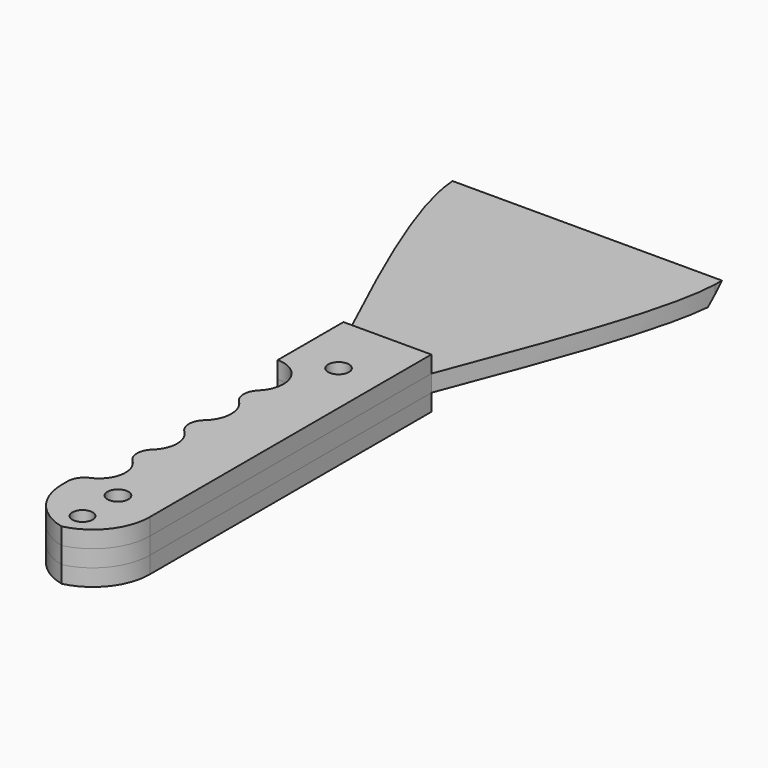
from build123d import *

# Parameters (mm, degrees)
F0_W         = 26.0835690424
F0_H         = 121.3984042406
F1_DEPTH     = 5
F2_T1_DEPTH  = 89.4974746831
F4_DEPTH     = 25
F5_T1_DEPTH  = 24.9013657706
F6_R         = 4.99999
F7_R         = 5
F8_T1_DEPTH  = 25.0040742563
F9_R         = 4.99999
F10_T1_DEPTH = 25.1951935832
F11_R        = 4.99999
F13_DEPTH    = 5
F15_DEPTH    = 5
F16_R        = 3.1
F17_DEPTH    = 25
F18_R        = 3
F19_DEPTH    = 25
F20_SIZE     = 4.99999


# Not quite as in the source:
# - a fillet or chamfer that OpenCascade refuses, or shapes differently, is made with other operations: its cross-section is extruded or revolved along the edge and cut away or added
# - a fillet or chamfer is up to 0.001 mm smaller than in the source, because OpenCascade refuses the exact size


with BuildPart() as f1:
    # F0 (on Top) → F1 (new body)
    with BuildSketch(Plane.XY):
        with BuildLine():
            Line((35.9049700201, 124.7347638011), (-44.0950299799, 124.7347638011))
            add(Edge.make_bspline(
                [(-13.5923651978, 46.1331680417), (-28.3171912792, 77.6195773739), (-43.0420173606, 109.1059867062), (-44.0950299799, 124.7347638011)],
                knots=[0, 0, 0, 0, 0.7080270969, 0.7080270969, 0.7080270969, 0.7080270969], degree=3))
            Line((-13.5923651978, 46.1331680417), (12.4912038445, 46.1331680417))
            add(Edge.make_bspline(
                [(12.4912038445, 46.1331680417), (23.8952472444, 75.9274680411), (35.2992906443, 105.7217680404), (35.9049700201, 122.1449805606)],
                knots=[0, 0, 0, 0, 0.6592241064, 0.6592241064, 0.6592241064, 0.6592241064], degree=3))
            Line((35.9049700201, 122.1449805606), (35.9049700201, 124.7347638011))
        make_face()
        with Locations((-0.5505806766, -14.5660340786)):
            Rectangle(F0_W, F0_H)
    extrude(amount=F1_DEPTH)

    # F2: fillet of radius 16.8994949366 on 2 edges, made by hand

    # F2_s2 → F2_t1 (cut)
    with BuildSketch(Plane.XY.offset(-42.2487373415)):
        with BuildLine():
            ThreePointArc((-13.5923651978, -58.3657412623), (-8.6426177295, -70.3154887306), (3.3071297388, -75.2652361989))
            Line((3.3071297388, -75.2652361989), (-13.5923651978, -75.2652361989))
            Line((-13.5923651978, -75.2652361989), (-13.5923651978, -58.3657412623))
        make_face()
        with BuildLine():
            ThreePointArc((-4.4082910921, -75.2652361989), (7.5414563762, -70.3154887306), (12.4912038445, -58.3657412623))
            Line((12.4912038445, -58.3657412623), (12.4912038445, -75.2652361989))
            Line((12.4912038445, -75.2652361989), (-4.4082910921, -75.2652361989))
        make_face()
    extrude(amount=F2_T1_DEPTH, mode=Mode.SUBTRACT)

    # F3 (on face) → F4 (cut)
    with BuildSketch(Plane.XY.offset(5)):
        with BuildLine():
            ThreePointArc((-13.5923651978, -52.2482340587), (-8.0995257077, -49.9730254459), (-5.8243170949, -44.4801859558))
            ThreePointArc((-5.8243170949, -44.4801859558), (-8.0995257077, -38.9873464656), (-13.5923651978, -36.7121378529))
            Line((-13.5923651978, -36.7121378529), (-13.5923651978, -52.2482340587))
        make_face()
        with BuildLine():
            Line((-13.5923651978, -17.6161278137), (-13.5923651978, -33.6357008568))
            ThreePointArc((-13.5923651978, -33.6357008568), (-7.9285908326, -31.2896887005), (-5.5825786763, -25.6259143353))
            ThreePointArc((-5.5825786763, -25.6259143353), (-7.9285908326, -19.96213997), (-13.5923651978, -17.6161278137))
        make_face()
        with BuildLine():
            Line((-13.5923651978, 2.3720021674), (-13.5923651978, -14.604575388))
            ThreePointArc((-13.5923651978, -14.604575388), (-7.5902386425, -12.1184131657), (-5.1040764201, -6.1162866103))
            ThreePointArc((-5.1040764201, -6.1162866103), (-7.5902386425, -0.1141600549), (-13.5923651978, 2.3720021674))
        make_face()
        with BuildLine():
            Line((-13.5923651978, 21.7131827375), (-13.5923651978, 4.5183054754))
            ThreePointArc((-13.5923651978, 4.5183054754), (-7.513058041, 7.0364369496), (-4.9949265668, 13.1157441065))
            ThreePointArc((-4.9949265668, 13.1157441065), (-7.513058041, 19.1950512633), (-13.5923651978, 21.7131827375))
        make_face()
    extrude(amount=-F4_DEPTH, mode=Mode.SUBTRACT)

    # F5: fillet of radius 5 on 1 edges, made by hand

    # F5_s2 → F5_t1 (cut)
    with BuildSketch(Plane.XY.offset(-9.9506828853)):
        with BuildLine():
            ThreePointArc((-10.5503778712, -37.3325370812), (-12.7631003469, -35.4895754009), (-13.5923651978, -32.7318646987))
            Line((-13.5923651978, -32.7318646987), (-13.5923651978, -36.7121378529))
            ThreePointArc((-13.5923651978, -36.7121378529), (-12.0400619013, -36.8688177604), (-10.5503778712, -37.3325370812))
        make_face()
    extrude(amount=F5_T1_DEPTH, mode=Mode.SUBTRACT)

    # F6 (radius 5 in the source; OpenCascade refuses exactly that, so slightly less here)
    f6_edges = [f1.edges().sort_by_distance(p)[0] for p in [
        (-13.510072, -33.635278, 2.5),
    ]]
    fillet(f6_edges, radius=F6_R)

    # F7
    f7_edges = [f1.edges().sort_by_distance(p)[0] for p in [
        (-13.592365, -52.248234, 2.5),
    ]]
    fillet(f7_edges, radius=F7_R)

    # F8: fillet of radius 5 on 1 edges, made by hand

    # F8_s2 → F8_t1 (cut)
    with BuildSketch(Plane.XY.offset(-10.0020371281)):
        with BuildLine():
            ThreePointArc((-10.5139954997, -18.2313000706), (-12.7521819912, -16.3894658503), (-13.5923651978, -13.6153129624))
            Line((-13.5923651978, -13.6153129624), (-13.5923651978, -17.6161278137))
            ThreePointArc((-13.5923651978, -17.6161278137), (-12.0227476565, -17.7714263892), (-10.5139954997, -18.2313000706))
        make_face()
    extrude(amount=F8_T1_DEPTH, mode=Mode.SUBTRACT)

    # F9 (radius 5 in the source; OpenCascade refuses exactly that, so slightly less here)
    f9_edges = [f1.edges().sort_by_distance(p)[0] for p in [
        (-13.49364, -14.604001, 2.5),
    ]]
    fillet(f9_edges, radius=F9_R)

    # F10: fillet of radius 5 on 1 edges, made by hand

    # F10_s2 → F10_t1 (cut)
    with BuildSketch(Plane.XY.offset(-10.0975967916)):
        with BuildLine():
            ThreePointArc((-10.4458249222, 1.7672614911), (-12.7316464532, 3.6063393511), (-13.5923651978, 6.411040884))
            Line((-13.5923651978, 6.411040884), (-13.5923651978, 2.3720021674))
            ThreePointArc((-13.5923651978, 2.3720021674), (-11.9903019195, 2.2194460885), (-10.4458249222, 1.7672614911))
        make_face()
    extrude(amount=F10_T1_DEPTH, mode=Mode.SUBTRACT)

    # F11 (radius 5 in the source; OpenCascade refuses exactly that, so slightly less here)
    f11_edges = [f1.edges().sort_by_distance(p)[0] for p in [
        (-13.223505, 4.526222, 2.5),
    ]]
    fillet(f11_edges, radius=F11_R)


with BuildPart() as f13:
    # F12 (on face) → F13 (new body)
    with BuildSketch(Plane.XY.offset(5)):
        with BuildLine():
            Line((12.4912038445, 46.1331680417), (-13.5923651978, 46.1331680417))
            Line((-13.5923651978, 46.1331680417), (-13.5923651978, 21.7131827375))
            ThreePointArc((-13.5923651978, 21.7131827375), (-5.6360261058, 16.3734456378), (-7.5628070571, 6.9870917553))
            add(Edge.make_bspline(
                [(-7.5911831215, -0.1132157245), (-7.7220544685, 0.0176144451), (-7.8479195294, 0.1550609527), (-7.9682435575, 0.2988565059), (-8.0825261727, 0.4486782277), (-8.1903056088, 0.604149631), (-8.3630630632, 0.8793988488), (-8.4314461626, 0.9966100443), (-8.4961606332, 1.1163214136), (-8.55706797, 1.2383679343), (-8.6140427893, 1.3625743295), (-8.7044044674, 1.5779889308), (-8.7398133996, 1.6682105076), (-8.7731600497, 1.7593543582), (-8.8044085072, 1.8513531954), (-8.8335265261, 1.9441378845), (-8.9259779929, 2.2647792954), (-8.9787300974, 2.4961463602), (-9.0183300846, 2.7307113036), (-9.0445030419, 2.9674123507), (-9.0571126109, 3.2051609509), (-9.0548218016, 3.7783711923), (-9.026462459, 4.1138191158), (-8.9710875527, 4.4460377153), (-8.889295394, 4.7719952295), (-8.7821710769, 5.0888005386), (-8.5974297226, 5.5195243383), (-8.5394639684, 5.6432713787), (-8.4775830857, 5.7648271817), (-8.4119138552, 5.8840174782), (-8.3425960964, 6.0006783584), (-8.1676441529, 6.274537971), (-8.0586255102, 6.4291429504), (-7.9431490529, 6.5780464502), (-7.8216795416, 6.7208756862), (-7.6947199209, 6.8573117912), (-7.5628070571, 6.9870917553)],
                knots=[0, 0, 0, 0, 0, 0, 0, 0.1452743272, 0.1452743272, 0.1452743272, 0.1452743272, 0.1452743272, 0.2488388047, 0.2488388047, 0.2488388047, 0.2488388047, 0.2488388047, 0.3220786555, 0.3220786555, 0.3220786555, 0.3220786555, 0.3220786555, 0.5000028667, 0.5000028667, 0.5000028667, 0.5000028667, 0.5000028667, 0.7511611873, 0.7511611873, 0.7511611873, 0.7511611873, 0.7511611873, 0.8547256681, 0.8547256681, 0.8547256681, 0.8547256681, 0.8547256681, 1, 1, 1, 1, 1, 1, 1], degree=6))
            ThreePointArc((-7.5911831215, -0.1132157245), (-5.1076987518, -6.3642415925), (-7.9519916275, -12.4595690698))
            add(Edge.make_bspline(
                [(-8.0741915729, -19.8201895772), (-8.2146874054, -19.6866523481), (-8.3498787146, -19.5457164219), (-8.4791425882, -19.397673153), (-8.6018965999, -19.242880944), (-8.7176036899, -19.0817628218), (-8.9020469019, -18.7970862585), (-8.9745726364, -18.6764633987), (-9.0431838813, -18.5531050443), (-9.1077251179, -18.4271925476), (-9.1680556762, -18.2989190025), (-9.2641399851, -18.0751050196), (-9.3020074648, -17.9806151083), (-9.3376061459, -17.8850944754), (-9.3708943601, -17.7886202923), (-9.4018347978, -17.6912719363), (-9.4999362532, -17.3541617447), (-9.5553644343, -17.1104852463), (-9.5962008224, -16.8632916711), (-9.6221316804, -16.6138110194), (-9.6330095305, -16.3633042906), (-9.6229942447, -15.7600411919), (-9.5872201159, -15.4074807738), (-9.5215801587, -15.0590267062), (-9.4268363554, -14.7181651477), (-9.3043198557, -14.3882045432), (-9.0957508169, -13.9436909497), (-9.0311955226, -13.8174907413), (-8.9625102443, -13.6937900517), (-8.8898419843, -13.572777199), (-8.8133521956, -13.4546282731), (-8.6195609158, -13.1762311036), (-8.498569346, -13.0190426179), (-8.3707447239, -12.8684104787), (-8.2366378556, -12.7247396524), (-8.0968427433, -12.5883690106), (-7.9519916275, -12.4595690698)],
                knots=[0, 0, 0, 0, 0, 0, 0, 0.1453888007, 0.1453888007, 0.1453888007, 0.1453888007, 0.1453888007, 0.2478981758, 0.2478981758, 0.2478981758, 0.2478981758, 0.2478981758, 0.3212921515, 0.3212921515, 0.3212921515, 0.3212921515, 0.3212921515, 0.5000035252, 0.5000035252, 0.5000035252, 0.5000035252, 0.5000035252, 0.7521018814, 0.7521018814, 0.7521018814, 0.7521018814, 0.7521018814, 0.8546112328, 0.8546112328, 0.8546112328, 0.8546112328, 0.8546112328, 1, 1, 1, 1, 1, 1, 1], degree=6))
            ThreePointArc((-8.0741915729, -19.8201895772), (-5.5829143759, -25.699246812), (-8.1814191878, -31.5317033086))
            add(Edge.make_bspline(
                [(-8.2453695343, -38.8452761337), (-8.384969873, -38.7128086357), (-8.5193466285, -38.5730441926), (-8.6478900937, -38.4262674837), (-8.770029703, -38.2728285149), (-8.8852388335, -38.1131402966), (-9.0689712626, -37.8311287667), (-9.1412284013, -37.7117140476), (-9.2096442684, -37.5895974592), (-9.2740664647, -37.4649555473), (-9.3343569472, -37.3379763089), (-9.4304900058, -37.1164646591), (-9.4684091329, -37.0229750356), (-9.5041042352, -36.9284632007), (-9.537534349, -36.833004192), (-9.5686627216, -36.736675206), (-9.6675382031, -36.4031780146), (-9.7237936262, -36.1621093417), (-9.765751421, -35.9175055055), (-9.7930987456, -35.6705620893), (-9.8056833842, -35.4225057442), (-9.8004571187, -34.8248127638), (-9.7680351894, -34.4752550097), (-9.7062685154, -34.1294690779), (-9.6158676256, -33.7908572209), (-9.4980971722, -33.4626544371), (-9.2965979244, -33.0197297642), (-9.2340962014, -32.8938242286), (-9.1675042686, -32.7703279126), (-9.0969634355, -32.6494263705), (-9.0226291652, -32.531293456), (-8.8339933533, -32.2525379377), (-8.7160094045, -32.0948887746), (-8.591205316, -31.9436090971), (-8.4601148523, -31.7991026439), (-8.3233146122, -31.6617093897), (-8.1814191878, -31.5317033086)],
                knots=[0, 0, 0, 0, 0, 0, 0, 0.1455538758, 0.1455538758, 0.1455538758, 0.1455538758, 0.1455538758, 0.2480776915, 0.2480776915, 0.2480776915, 0.2480776915, 0.2480776915, 0.3214424039, 0.3214424039, 0.3214424039, 0.3214424039, 0.3214424039, 0.5000033945, 0.5000033945, 0.5000033945, 0.5000033945, 0.5000033945, 0.7519223516, 0.7519223516, 0.7519223516, 0.7519223516, 0.7519223516, 0.8544461495, 0.8544461495, 0.8544461495, 0.8544461495, 0.8544461495, 1, 1, 1, 1, 1, 1, 1], degree=6))
            ThreePointArc((-8.2453695343, -38.8452761337), (-5.9476146715, -45.8587216712), (-10.5503778712, -51.6278348303))
            ThreePointArc((-10.5503778712, -51.6278348303), (-12.7631003469, -53.4707965107), (-13.5923651978, -56.2285072128))
            Line((-13.5923651978, -56.2285072128), (-13.5923651978, -58.3657412623))
            ThreePointArc((-13.5923651978, -58.3657412623), (-9.9364779031, -68.8633498347), (-0.5505806767, -74.8190387878))
            ThreePointArc((-0.5505806767, -74.8190387878), (8.8353165498, -68.8633498347), (12.4912038445, -58.3657412623))
            Line((12.4912038445, -58.3657412623), (12.4912038445, 46.1331680417))
        make_face()
    extrude(amount=F13_DEPTH)


with BuildPart() as f15:
    # F14 (on face) → F15 (new body)
    with BuildSketch(Plane(origin=(0, 0, 0), x_dir=(1, 0, 0), z_dir=(0, 0, -1))):
        with BuildLine():
            Line((-13.5923651978, -46.1331680417), (12.4912038445, -46.1331680417))
            Line((12.4912038445, -46.1331680417), (12.4912038445, 58.3657412623))
            ThreePointArc((12.4912038445, 58.3657412623), (8.8353165498, 68.8633498347), (-0.5505806767, 74.8190387878))
            ThreePointArc((-0.5505806767, 74.8190387878), (-9.9364779031, 68.8633498347), (-13.5923651978, 58.3657412623))
            Line((-13.5923651978, 58.3657412623), (-13.5923651978, 56.2285072128))
            ThreePointArc((-13.5923651978, 56.2285072128), (-12.7631003469, 53.4707965107), (-10.5503778712, 51.6278348303))
            ThreePointArc((-10.5503778712, 51.6278348303), (-5.9476146715, 45.8587216712), (-8.2453695343, 38.8452761337))
            add(Edge.make_bspline(
                [(-8.2453695343, 38.8452761337), (-8.384969873, 38.7128086357), (-8.5193466285, 38.5730441926), (-8.6478900937, 38.4262674837), (-8.770029703, 38.2728285149), (-8.8852388335, 38.1131402966), (-9.0689712626, 37.8311287667), (-9.1412284013, 37.7117140476), (-9.2096442684, 37.5895974592), (-9.2740664647, 37.4649555473), (-9.3343569472, 37.3379763089), (-9.4304900058, 37.1164646591), (-9.4684091329, 37.0229750356), (-9.5041042352, 36.9284632007), (-9.537534349, 36.833004192), (-9.5686627216, 36.736675206), (-9.6675382031, 36.4031780146), (-9.7237936262, 36.1621093417), (-9.765751421, 35.9175055055), (-9.7930987456, 35.6705620893), (-9.8056833842, 35.4225057442), (-9.8004571187, 34.8248127638), (-9.7680351894, 34.4752550097), (-9.7062685154, 34.1294690779), (-9.6158676256, 33.7908572209), (-9.4980971722, 33.4626544371), (-9.2965979244, 33.0197297642), (-9.2340962014, 32.8938242286), (-9.1675042686, 32.7703279126), (-9.0969634355, 32.6494263705), (-9.0226291652, 32.531293456), (-8.8339933533, 32.2525379377), (-8.7160094045, 32.0948887746), (-8.591205316, 31.9436090971), (-8.4601148523, 31.7991026439), (-8.3233146122, 31.6617093897), (-8.1814191878, 31.5317033086)],
                knots=[0, 0, 0, 0, 0, 0, 0, 0.1455538758, 0.1455538758, 0.1455538758, 0.1455538758, 0.1455538758, 0.2480776915, 0.2480776915, 0.2480776915, 0.2480776915, 0.2480776915, 0.3214424039, 0.3214424039, 0.3214424039, 0.3214424039, 0.3214424039, 0.5000033945, 0.5000033945, 0.5000033945, 0.5000033945, 0.5000033945, 0.7519223516, 0.7519223516, 0.7519223516, 0.7519223516, 0.7519223516, 0.8544461495, 0.8544461495, 0.8544461495, 0.8544461495, 0.8544461495, 1, 1, 1, 1, 1, 1, 1], degree=6))
            ThreePointArc((-8.1814191878, 31.5317033086), (-5.5829143759, 25.699246812), (-8.0741915729, 19.8201895772))
            add(Edge.make_bspline(
                [(-8.0741915729, 19.8201895772), (-8.2146874054, 19.6866523481), (-8.3498787146, 19.5457164219), (-8.4791425882, 19.397673153), (-8.6018965999, 19.242880944), (-8.7176036899, 19.0817628218), (-8.9020469019, 18.7970862585), (-8.9745726364, 18.6764633987), (-9.0431838813, 18.5531050443), (-9.1077251179, 18.4271925476), (-9.1680556762, 18.2989190025), (-9.2641399851, 18.0751050196), (-9.3020074648, 17.9806151083), (-9.3376061459, 17.8850944754), (-9.3708943601, 17.7886202923), (-9.4018347978, 17.6912719363), (-9.4999362532, 17.3541617447), (-9.5553644343, 17.1104852463), (-9.5962008224, 16.8632916711), (-9.6221316804, 16.6138110194), (-9.6330095305, 16.3633042906), (-9.6229942447, 15.7600411919), (-9.5872201159, 15.4074807738), (-9.5215801587, 15.0590267062), (-9.4268363554, 14.7181651477), (-9.3043198557, 14.3882045432), (-9.0957508169, 13.9436909497), (-9.0311955226, 13.8174907413), (-8.9625102443, 13.6937900517), (-8.8898419843, 13.572777199), (-8.8133521956, 13.4546282731), (-8.6195609158, 13.1762311036), (-8.498569346, 13.0190426179), (-8.3707447239, 12.8684104787), (-8.2366378556, 12.7247396524), (-8.0968427433, 12.5883690106), (-7.9519916275, 12.4595690698)],
                knots=[0, 0, 0, 0, 0, 0, 0, 0.1453888007, 0.1453888007, 0.1453888007, 0.1453888007, 0.1453888007, 0.2478981758, 0.2478981758, 0.2478981758, 0.2478981758, 0.2478981758, 0.3212921515, 0.3212921515, 0.3212921515, 0.3212921515, 0.3212921515, 0.5000035252, 0.5000035252, 0.5000035252, 0.5000035252, 0.5000035252, 0.7521018814, 0.7521018814, 0.7521018814, 0.7521018814, 0.7521018814, 0.8546112328, 0.8546112328, 0.8546112328, 0.8546112328, 0.8546112328, 1, 1, 1, 1, 1, 1, 1], degree=6))
            ThreePointArc((-7.9519916275, 12.4595690698), (-5.1076987518, 6.3642415925), (-7.5911831215, 0.1132157245))
            add(Edge.make_bspline(
                [(-7.5911831215, 0.1132157245), (-7.7220544685, -0.0176144451), (-7.8479195294, -0.1550609527), (-7.9682435575, -0.2988565059), (-8.0825261727, -0.4486782277), (-8.1903056088, -0.604149631), (-8.3630630632, -0.8793988488), (-8.4314461626, -0.9966100443), (-8.4961606332, -1.1163214136), (-8.55706797, -1.2383679343), (-8.6140427893, -1.3625743295), (-8.7044044674, -1.5779889308), (-8.7398133996, -1.6682105076), (-8.7731600497, -1.7593543582), (-8.8044085072, -1.8513531954), (-8.8335265261, -1.9441378845), (-8.9259779929, -2.2647792954), (-8.9787300974, -2.4961463602), (-9.0183300846, -2.7307113036), (-9.0445030419, -2.9674123507), (-9.0571126109, -3.2051609509), (-9.0548218016, -3.7783711923), (-9.026462459, -4.1138191158), (-8.9710875527, -4.4460377153), (-8.889295394, -4.7719952295), (-8.7821710769, -5.0888005386), (-8.5974297226, -5.5195243383), (-8.5394639684, -5.6432713787), (-8.4775830857, -5.7648271817), (-8.4119138552, -5.8840174782), (-8.3425960964, -6.0006783584), (-8.1676441529, -6.274537971), (-8.0586255102, -6.4291429504), (-7.9431490529, -6.5780464502), (-7.8216795416, -6.7208756862), (-7.6947199209, -6.8573117912), (-7.5628070571, -6.9870917553)],
                knots=[0, 0, 0, 0, 0, 0, 0, 0.1452743272, 0.1452743272, 0.1452743272, 0.1452743272, 0.1452743272, 0.2488388047, 0.2488388047, 0.2488388047, 0.2488388047, 0.2488388047, 0.3220786555, 0.3220786555, 0.3220786555, 0.3220786555, 0.3220786555, 0.5000028667, 0.5000028667, 0.5000028667, 0.5000028667, 0.5000028667, 0.7511611873, 0.7511611873, 0.7511611873, 0.7511611873, 0.7511611873, 0.8547256681, 0.8547256681, 0.8547256681, 0.8547256681, 0.8547256681, 1, 1, 1, 1, 1, 1, 1], degree=6))
            ThreePointArc((-7.5628070571, -6.9870917553), (-5.6360261058, -16.3734456378), (-13.5923651978, -21.7131827375))
            Line((-13.5923651978, -21.7131827375), (-13.5923651978, -46.1331680417))
        make_face()
    extrude(amount=F15_DEPTH)


with BuildPart() as f17_tool:
    # F16 (on face) → F17 (new body)
    with BuildSketch(Plane.XY.offset(10)):
        with Locations((0, -54.5530170202)):
            Circle(F16_R)
        with Locations((0, 27.3210182786)):
            Circle(F16_R)
    extrude(amount=-F17_DEPTH)


with BuildPart() as f1_1:
    add(f1.part)

    # F17: cut by f17_tool
    add(f17_tool.part, mode=Mode.SUBTRACT)


with BuildPart() as f13_1:
    add(f13.part)

    # F17: cut by f17_tool
    add(f17_tool.part, mode=Mode.SUBTRACT)


with BuildPart() as f15_1:
    add(f15.part)

    # F17: cut by f17_tool
    add(f17_tool.part, mode=Mode.SUBTRACT)


with BuildPart() as f19_tool:
    # F18 (on face) → F19 (new body)
    with BuildSketch(Plane.XY.offset(10)):
        with Locations((0, -67.7251815796)):
            Circle(F18_R)
    extrude(amount=-F19_DEPTH)


with BuildPart() as f1_2:
    add(f1_1.part)

    # F19: cut by f19_tool
    add(f19_tool.part, mode=Mode.SUBTRACT)

    # F20 (size 5 in the source; OpenCascade refuses exactly that, so slightly less here)
    f20_edges = [f1_2.edges().sort_by_distance(p)[0] for p in [
        (-4.09503, 124.734764, 0),
    ]]
    chamfer(f20_edges, length=F20_SIZE)


with BuildPart() as f13_2:
    add(f13_1.part)

    # F19: cut by f19_tool
    add(f19_tool.part, mode=Mode.SUBTRACT)


with BuildPart() as f15_2:
    add(f15_1.part)

    # F19: cut by f19_tool
    add(f19_tool.part, mode=Mode.SUBTRACT)


solid = Compound([f1_2.part, f13_2.part, f15_2.part])
